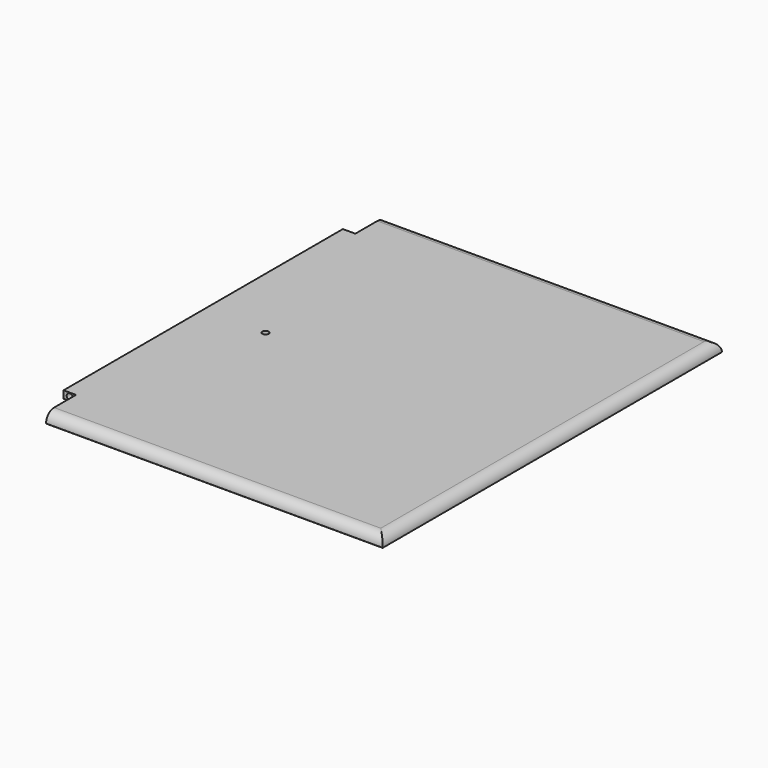
from build123d import *

# Parameters (mm, degrees)
F1_DEPTH    = 6.35
F0_W        = 6.35
F0_H        = 177.8
F2_DEPTH    = 3.81
F3_R        = 1.5875
F4_DEPTH    = 177.8
F5_R        = 1.5875
F6_DEPTH    = 6.35
F7_R        = 5.08
F8_T1_DEPTH = 232.7005208253
F8_T3_DEPTH = 188.2505208253


# Not quite as in the source:
# - a fillet or chamfer that OpenCascade refuses, or shapes differently, is made with other operations: its cross-section is extruded or revolved along the edge and cut away or added


with BuildPart() as f1:
    # F0 (on Top) → F1 (new body)
    with BuildSketch(Plane.XY):
        Polygon((-11.6160511255, 102.6400476694), (-11.6160511255, -75.1599523306), (-11.6160511255, -94.2099523306), (159.8339488745, -94.2099523306), (159.8339488745, 121.6900476694), (-11.6160511255, 121.6900476694), align=None)
    extrude(amount=-F1_DEPTH)

    # F0 (on Top) → F2 (join)
    with BuildSketch(Plane.XY):
        with Locations((-14.7910511255, 13.7400476694)):
            Rectangle(F0_W, F0_H)
    extrude(amount=-F2_DEPTH)

    # F3 (on face) → F4 (cut)
    with BuildSketch(Plane.XZ.offset(75.1599523306)):
        with Locations((-14.7910511255, -1.905)):
            Circle(F3_R)
    extrude(amount=-F4_DEPTH, mode=Mode.SUBTRACT)

    # F5 (on face) → F6 (cut)
    with BuildSketch(Plane.XY):
        with Locations((13.7839488745, 13.7400476694)):
            Circle(F5_R)
    extrude(amount=-F6_DEPTH, mode=Mode.SUBTRACT)

    # F7
    f7_edges = [f1.edges().sort_by_distance(p)[0] for p in [
        (74.108949, -94.209952, 0),
        (159.833949, 13.740048, 0),
        (74.108949, 121.690048, 0),
    ]]
    fillet(f7_edges, radius=F7_R)

    # F8: fillet of radius 5.08 on 3 edges, made by hand

    # F8_s2 → F8_t1 (cut)
    with BuildSketch(Plane.XZ.offset(-130.090308082)):
        with BuildLine():
            ThreePointArc((156.4738447094, -6.35), (158.2698959336, -6.0219048812), (159.8339488745, -5.08))
            Line((159.8339488745, -5.08), (159.8339488745, -6.35))
            Line((159.8339488745, -6.35), (156.4738447094, -6.35))
        make_face()
    extrude(amount=F8_T1_DEPTH, mode=Mode.SUBTRACT)

    # F8_s4 → F8_t3 (cut)
    with BuildSketch(Plane.YZ.offset(-20.0163115382)):
        with BuildLine():
            ThreePointArc((-90.8498481655, -6.35), (-92.6458993898, -6.0219048812), (-94.2099523306, -5.08))
            Line((-94.2099523306, -5.08), (-94.2099523306, -6.35))
            Line((-94.2099523306, -6.35), (-90.8498481655, -6.35))
        make_face()
        with BuildLine():
            ThreePointArc((121.6900476694, -5.08), (120.1259947286, -6.0219048812), (118.3299435044, -6.35))
            Line((118.3299435044, -6.35), (121.6900476694, -6.35))
            Line((121.6900476694, -6.35), (121.6900476694, -5.08))
        make_face()
    extrude(amount=F8_T3_DEPTH, mode=Mode.SUBTRACT)


solid = f1.part
